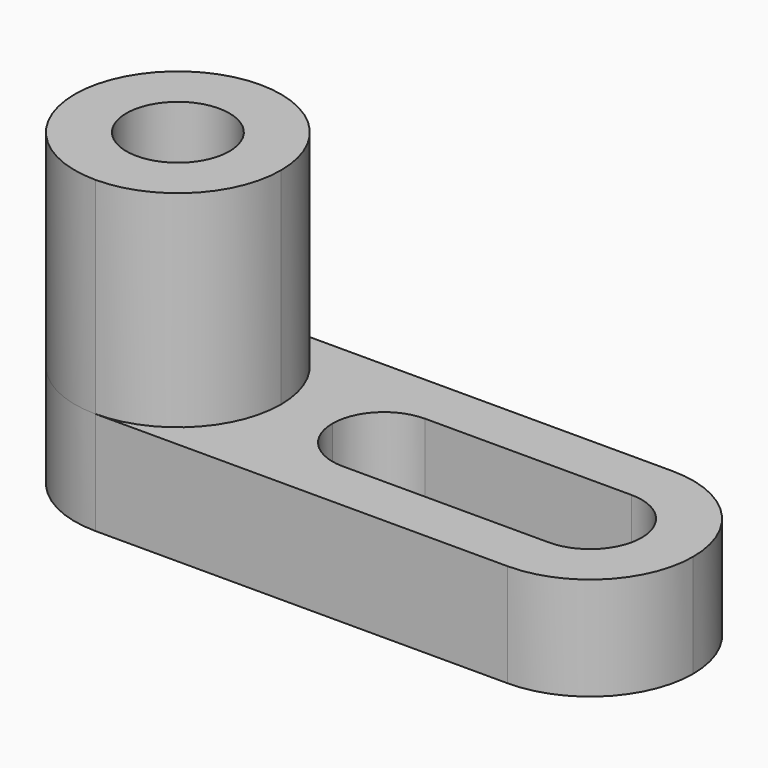
from build123d import *

# Parameters (mm, degrees)
F0_W     = 76.2
F0_H     = 12.7
F1_DEPTH = 25.4
F3_DEPTH = 12.7
F4_R     = 6.35
F5_DEPTH = 25.4


# Not quite as in the source:
# - ends of sketch curves that miss each other by under 0.0002 mm in the source are joined


with BuildPart() as f1:
    # F0 (on Front) → F1 (new body)
    with BuildSketch(Plane.XZ):
        with Locations((38.1, 6.35)):
            Rectangle(F0_W, F0_H)
    extrude(amount=F1_DEPTH)

    # F2 (on face) → F3 (cut)
    with BuildSketch(Plane.XY.offset(12.7)):
        with BuildLine():
            Line((0, -25.4), (12.7, -25.4))
            ThreePointArc((12.7, -25.4), (3.7197438789, -21.6802561211), (0, -12.7))
            Line((0, -12.7), (0, -25.4))
        make_face()
        with BuildLine():
            ThreePointArc((0, -12.7), (3.7197438789, -3.7197438789), (12.7, 0))
            Line((12.7, 0), (0, 0))
            Line((0, 0), (0, -12.7))
        make_face()
        with BuildLine():
            ThreePointArc((63.5, -19.05), (57.15, -12.7), (63.5, -6.35))
            Line((63.5, -6.35), (38.0999993506, -6.35))
            ThreePointArc((38.0999993506, -6.35), (42.5901278309, -8.2098717099), (44.45, -12.7))
            ThreePointArc((44.45, -12.7), (42.5901280605, -17.1901280605), (38.1, -19.05))
            Line((38.1, -19.05), (63.5, -19.05))
        make_face()
        with BuildLine():
            Line((38.0999996753, -12.7), (38.0999993506, -6.35))
            ThreePointArc((38.0999993506, -6.35), (33.6098717099, -8.2098721691), (31.75, -12.7))
            Line((31.75, -12.7), (38.0999996753, -12.7))
        make_face()
        with BuildLine():
            ThreePointArc((31.75, -12.7), (33.6098719395, -17.1901280605), (38.1, -19.05))
            Line((38.1, -19.05), (38.0999996753, -12.7))
            Line((38.0999996753, -12.7), (31.75, -12.7))
        make_face()
        with BuildLine():
            ThreePointArc((44.45, -12.7), (42.5901278309, -8.2098717099), (38.0999993506, -6.35))
            Line((38.0999993506, -6.35), (38.0999996753, -12.7))
            Line((38.0999996753, -12.7), (38.1, -19.05))
            ThreePointArc((38.1, -19.05), (42.5901280605, -17.1901280605), (44.45, -12.7))
        make_face()
        with BuildLine():
            Line((63.5, -19.05), (63.5, -6.35))
            ThreePointArc((63.5, -6.35), (57.15, -12.7), (63.5, -19.05))
        make_face()
        with BuildLine():
            ThreePointArc((63.5, -19.05), (67.9901280605, -17.1901280605), (69.85, -12.7))
            ThreePointArc((69.85, -12.7), (67.9901280605, -8.2098719395), (63.5, -6.35))
            Line((63.5, -6.35), (63.5, -19.05))
        make_face()
        with BuildLine():
            Line((76.2, 0), (63.5, 0))
            ThreePointArc((63.5, 0), (72.4802561211, -3.7197438789), (76.2, -12.7))
            Line((76.2, -12.7), (76.2, 0))
        make_face()
        with BuildLine():
            ThreePointArc((76.2, -12.7), (72.4802561211, -21.6802561211), (63.5, -25.4))
            Line((63.5, -25.4), (76.2, -25.4))
            Line((76.2, -25.4), (76.2, -12.7))
        make_face()
    extrude(amount=-F3_DEPTH, mode=Mode.SUBTRACT)

    # F4 (on face) → F5 (join)
    with BuildSketch(Plane.XY.offset(12.7)):
        with BuildLine():
            ThreePointArc((12.7, -25.4), (21.6802561211, -21.6802561211), (25.4, -12.7))
            ThreePointArc((25.4, -12.7), (21.6802561211, -3.7197438789), (12.7, 0))
            ThreePointArc((12.7, 0), (0, -12.7), (12.7, -25.4))
        make_face()
        with Locations((12.7, -12.7)):
            Circle(F4_R, mode=Mode.SUBTRACT)
    extrude(amount=F5_DEPTH)


solid = f1.part
